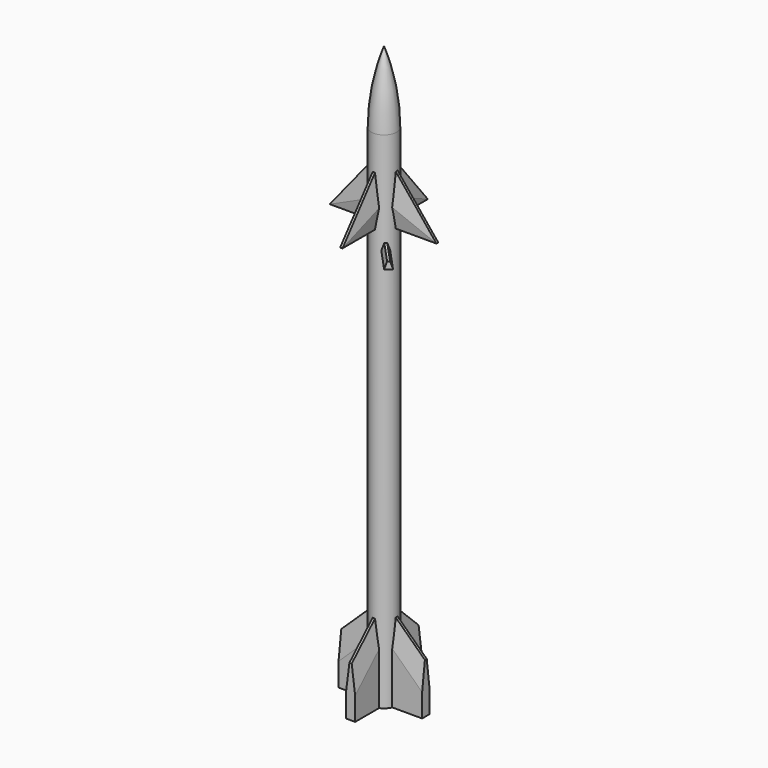
from build123d import *

# Parameters (mm, degrees)
F3_DEPTH     = 0.2
F4_C1_SIZE2  = 0.15
F4_C1_SIZE   = 0.8506922729
F4_C2_SIZE2  = 0.8506922729
F4_C2_SIZE   = 0.15
F4_C3_SIZE2  = 0.15
F4_C3_SIZE   = 0.8506922729
F4_C4_SIZE2  = 0.8506922729
F4_C4_SIZE   = 0.15
F4_C5_SIZE2  = 0.8506922729
F4_C5_SIZE   = 0.15
F4_C6_SIZE2  = 0.15
F4_C6_SIZE   = 0.8506922729
F5_T4_DEPTH  = 5.1346986834
F5_S5_R      = 0.5555555556
F5_T6_DEPTH  = 4
F5_T10_DEPTH = 5.1346986834
F5_S11_R     = 0.5555555556
F5_T12_DEPTH = 4
F6_T4_DEPTH  = 6.228597395
F6_S5_R      = 0.5555555556
F6_T6_DEPTH  = 5
F6_T10_DEPTH = 6.228597395
F6_S11_R     = 0.5555555556
F6_T12_DEPTH = 5
F6_T16_DEPTH = 6.2002452754
F6_S17_R     = 0.5555555556
F6_T18_DEPTH = 5
F6_T22_DEPTH = 5.055252599
F6_S23_R     = 0.5555555556
F6_T24_DEPTH = 4
F7_COUNT     = 4
F10_DEPTH    = 0.15
F11_SIZE2    = 0.2747477419
F11_SIZE     = 0.1
F11_2_SIZE2  = 0.2747477419
F11_2_SIZE   = 0.1
F12_SIZE2    = 0.2747477419
F12_SIZE     = 0.1


# Not quite as in the source:
# - a fillet or chamfer that OpenCascade refuses, or shapes differently, is made with other operations: its cross-section is extruded or revolved along the edge and cut away or added


with BuildPart() as f1:
    # F0 (on Front) → F1 (revolve)
    with BuildSketch(Plane.XZ):
        with BuildLine():
            Line((0, 25.1388888889), (0, 0))
            Line((0, 0), (0.5555555556, 0))
            Line((0.5555555556, 0), (0.5555555556, 22.0138888889))
            ThreePointArc((0.5555555556, 22.0138888889), (0.4155862794, 23.6008881781), (0, 25.1388888889))
        make_face()
    revolve(axis=Axis((0, 0, 12.5694444444), (0, 0, 1)))

    # F2 (on Front) → F3 (join, symmetric)
    with BuildSketch(Plane.XZ):
        Polygon((0.25, 20.8982843137), (-0.25, 20.8982843137), (-2.3263888889, 18.3333333333), (2.3263888889, 18.3333333333), align=None)
        Polygon((-0.5555555556, 0), (0.5555555556, 0), (1.8229166667, 0), (1.8229166667, 2.1875), (0.25, 3.6957762557), (-0.25, 3.6957762557), (-1.8229166667, 2.1875), (-1.8229166667, 0), align=None)
    extrude(amount=F3_DEPTH, both=True)

    # F4: chamfer of 0.15 x 0.8506922729 on 6 edges, made by hand

    # F4_c1
    f4_c1_edges = [f1.edges().sort_by_distance(p)[0] for p in [
        (1.1706117509, -0.2, 2.8129978645),
    ]]
    f4_c1_side = f1.faces().sort_by_distance((1.1685353906, -0.2, 2.8108325173))[0]
    chamfer(f4_c1_edges, length=F4_C1_SIZE, length2=F4_C1_SIZE2, reference=f4_c1_side)

    # F4_c2
    f4_c2_edges = [f1.edges().sort_by_distance(p)[0] for p in [
        (-1.1706117509, 0.2, 2.8129978645),
    ]]
    f4_c2_side = f1.faces().sort_by_distance((-1.1706117509, 0.197, 2.8129978645))[0]
    chamfer(f4_c2_edges, length=F4_C2_SIZE, length2=F4_C2_SIZE2, reference=f4_c2_side)

    # F4_c3
    f4_c3_edges = [f1.edges().sort_by_distance(p)[0] for p in [
        (1.422347862, 0.2, 19.450089896),
    ]]
    f4_c3_side = f1.faces().sort_by_distance((1.4200161274, 0.2, 19.4482023013))[0]
    chamfer(f4_c3_edges, length=F4_C3_SIZE, length2=F4_C3_SIZE2, reference=f4_c3_side)

    # F4_c4
    f4_c4_edges = [f1.edges().sort_by_distance(p)[0] for p in [
        (1.422347862, -0.2, 19.450089896),
    ]]
    f4_c4_side = f1.faces().sort_by_distance((1.422347862, -0.197, 19.450089896))[0]
    chamfer(f4_c4_edges, length=F4_C4_SIZE, length2=F4_C4_SIZE2, reference=f4_c4_side)

    # F4_c5
    f4_c5_edges = [f1.edges().sort_by_distance(p)[0] for p in [
        (-1.422347862, -0.2, 18.3333333333),
    ]]
    f4_c5_side = f1.faces().sort_by_distance((-1.422347862, -0.197, 18.3333333333))[0]
    chamfer(f4_c5_edges, length=F4_C5_SIZE, length2=F4_C5_SIZE2, reference=f4_c5_side)

    # F4_c6
    f4_c6_edges = [f1.edges().sort_by_distance(p)[0] for p in [
        (-1.0780200372, -0.2, 19.8754360324),
    ]]
    f4_c6_side = f1.faces().sort_by_distance((-1.0756883026, -0.2, 19.8735484378))[0]
    chamfer(f4_c6_edges, length=F4_C6_SIZE, length2=F4_C6_SIZE2, reference=f4_c6_side)

    # F5: chamfer of 0.15 x 0.8506922729 on 2 edges, made by hand


with BuildPart() as f5_tool2:
    # F5_s3 → F5_t4 (new body)
    with BuildSketch(Plane.YZ.offset(-1.69225004)):
        Polygon((-0.2, 19.1840256063), (-0.05, 18.3333333333), (-0.2, 18.3333333333), align=None)
    extrude(amount=F5_T4_DEPTH)

    # F5_s5 → F5_t6 (cut, symmetric)
    with BuildSketch(Plane.XY.offset(18.8)):
        Circle(F5_S5_R)
    extrude(amount=F5_T6_DEPTH, both=True, mode=Mode.SUBTRACT)


with BuildPart() as f1_1:
    add(f1.part)

    # F5_t1: cut F5_tool2
    add(f5_tool2.part, mode=Mode.SUBTRACT)


with BuildPart() as f5_tool8:
    # F5_s9 → F5_t10 (new body)
    with BuildSketch(Plane.YZ.offset(-1.69225004)):
        Polygon((0.05, 18.3333333333), (0.2, 19.1840256063), (0.2, 18.3333333333), align=None)
    extrude(amount=F5_T10_DEPTH)

    # F5_s11 → F5_t12 (cut, symmetric)
    with BuildSketch(Plane.XY.offset(18.8)):
        Circle(F5_S11_R)
    extrude(amount=F5_T12_DEPTH, both=True, mode=Mode.SUBTRACT)


with BuildPart() as f1_2:
    add(f1_1.part)

    # F5_t7: cut F5_tool8
    add(f5_tool8.part, mode=Mode.SUBTRACT)

    # F6: chamfer of 0.15 x 0.8506922729 on 4 edges, made by hand


with BuildPart() as f6_tool2:
    # F6_s3 → F6_t4 (new body)
    with BuildSketch(Plane(origin=(1.4524378373, 0, -1.3927486111), x_dir=(0, 1, 0), z_dir=(-0.7217823715, 0, 0.6921200822))):
        Polygon((0.05, -2.8405761708), (0.2, -1.9898838979), (0.2, -2.8405761708), align=None)
    extrude(amount=F6_T4_DEPTH)

    # F6_s5 → F6_t6 (cut, symmetric)
    with BuildSketch(Plane.XY.offset(2.5)):
        Circle(F6_S5_R)
    extrude(amount=F6_T6_DEPTH, both=True, mode=Mode.SUBTRACT)


with BuildPart() as f1_3:
    add(f1_2.part)

    # F6_t1: cut F6_tool2
    add(f6_tool2.part, mode=Mode.SUBTRACT)


with BuildPart() as f6_tool8:
    # F6_s9 → F6_t10 (new body)
    with BuildSketch(Plane(origin=(3.0432539614, 0, 2.9181887301), x_dir=(0, 1, 0), z_dir=(-0.7217823715, 0, -0.6921200822))):
        Polygon((-0.2, -1.9898838979), (-0.05, -2.8405761708), (-0.2, -2.8405761708), align=None)
    extrude(amount=F6_T10_DEPTH)

    # F6_s11 → F6_t12 (cut, symmetric)
    with BuildSketch(Plane.XY.offset(2.5)):
        Circle(F6_S11_R)
    extrude(amount=F6_T12_DEPTH, both=True, mode=Mode.SUBTRACT)


with BuildPart() as f1_4:
    add(f1_3.part)

    # F6_t7: cut F6_tool8
    add(f6_tool8.part, mode=Mode.SUBTRACT)


with BuildPart() as f6_tool14:
    # F6_s15 → F6_t16 (new body)
    with BuildSketch(Plane(origin=(11.2437188953, 0, 13.8892998119), x_dir=(0, 1, 0), z_dir=(-0.6291982287, 0, -0.7772448707))):
        Polygon((0.05, -13.3434746901), (0.2, -12.4927824171), (0.2, -13.3434746901), align=None)
    extrude(amount=F6_T16_DEPTH)

    # F6_s17 → F6_t18 (cut, symmetric)
    with BuildSketch(Plane.XY.offset(19.6)):
        Circle(F6_S17_R)
    extrude(amount=F6_T18_DEPTH, both=True, mode=Mode.SUBTRACT)


with BuildPart() as f1_5:
    add(f1_4.part)

    # F6_t13: cut F6_tool14
    add(f6_tool14.part, mode=Mode.SUBTRACT)


with BuildPart() as f6_tool20:
    # F6_s21 → F6_t22 (new body)
    with BuildSketch(Plane.YZ.offset(-4.5369457639)):
        Polygon((0.05, 18.3333333333), (0.2, 19.1840256063), (0.2, 18.3333333333), align=None)
    extrude(amount=F6_T22_DEPTH)

    # F6_s23 → F6_t24 (cut, symmetric)
    with BuildSketch(Plane.XY.offset(18.8)):
        Circle(F6_S23_R)
    extrude(amount=F6_T24_DEPTH, both=True, mode=Mode.SUBTRACT)


with BuildPart() as f1_6:
    add(f1_5.part)

    # F6_t19: cut F6_tool20
    add(f6_tool20.part, mode=Mode.SUBTRACT)


with BuildPart() as f7_1:
    # F7: instance of F1
    add(f1_6.part.rotate(Axis((0, 0, 0), (0, 0, 1)), 1 * 360 / F7_COUNT))


with BuildPart() as f7_2:
    # F7: instance of F1
    add(f1_6.part.rotate(Axis((0, 0, 0), (0, 0, 1)), 2 * 360 / F7_COUNT))


with BuildPart() as f7_3:
    # F7: instance of F1
    add(f1_6.part.rotate(Axis((0, 0, 0), (0, 0, 1)), 3 * 360 / F7_COUNT))


with BuildPart() as f1_7:
    add(f1_6.part)

    add(f7_1.part)  # F10 merges F7_1

    add(f7_2.part)  # F10 merges F7_2

    add(f7_3.part)  # F10 merges F7_3
    # F9 (on face) → F10 (join, symmetric)
    with BuildSketch(Plane(origin=(0, 0, 0), x_dir=(0.7071067812, -0.7071067812, 0), z_dir=(-0.7071067812, -0.7071067812, 0))):
        Polygon((0.25, 17.9613043319), (-0.25, 17.9613043319), (-1.4106974118, 17.6041666667), (-1.4106974118, 17.2916666667), (-0.25, 17.6488043319), (0.25, 17.6488043319), (1.4106974118, 17.2916666667), (1.4106974118, 17.6041666667), align=None)
    extrude(amount=F10_DEPTH, both=True)

    # F11
    f11_edges = [f1_7.edges().sort_by_distance(p)[0] for p in [
        (0.581814, -0.793946, 17.738901),
        (0.793946, -0.581814, 17.738901),
    ]]
    f11_side = f1_7.faces().sort_by_distance((0.692747, -0.692747, 17.736784))[0]
    chamfer(f11_edges, length=F11_SIZE, length2=F11_SIZE2, reference=f11_side)

    # F11#2
    f11_2_edges = [f1_7.edges().sort_by_distance(p)[0] for p in [
        (-0.793946, 0.581814, 17.738901),
    ]]
    f11_2_side = f1_7.faces().sort_by_distance((-0.692747, 0.692747, 17.736784))[0]
    chamfer(f11_2_edges, length=F11_2_SIZE, length2=F11_2_SIZE2, reference=f11_2_side)

    # F12
    f12_edges = [f1_7.edges().sort_by_distance(p)[0] for p in [
        (-0.581814, 0.793946, 17.738901),
    ]]
    f12_side = f1_7.faces().sort_by_distance((-0.657679, 0.72889, 17.73655))[0]
    chamfer(f12_edges, length=F12_SIZE, length2=F12_SIZE2, reference=f12_side)


solid = f1_7.part
